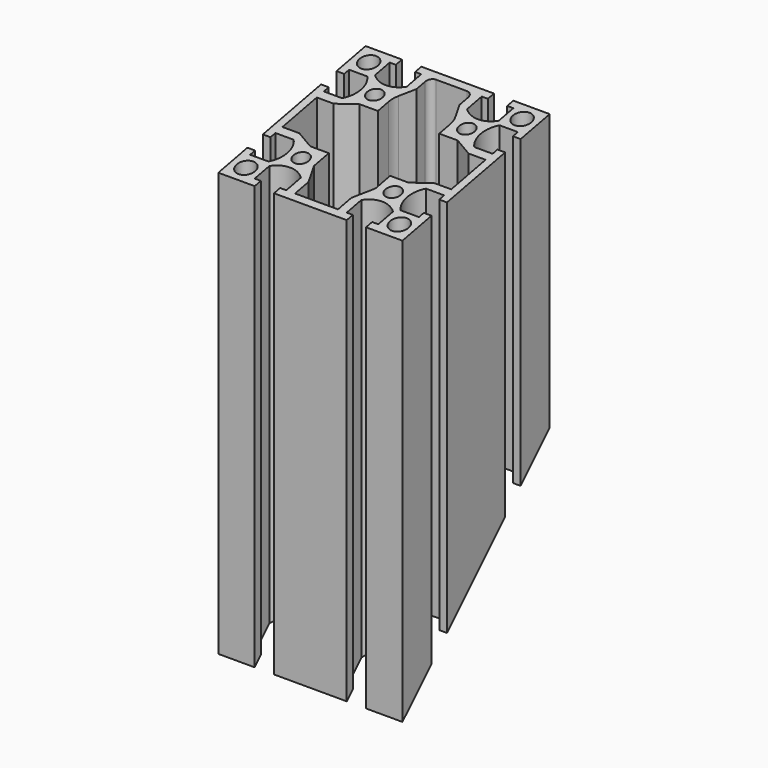
from build123d import *

# Parameters (mm, degrees)
F0_R          = 3
F0_R_2        = 2.5
F1_DEPTH      = 150
F2_R          = 2
F3_R          = 7
F6_DEPTH      = 30
F6_DEPTH_BACK = 30


# Not quite as in the source:
# - a feature names something its author has since deleted; it is built from what else it names


with BuildPart() as f1:
    # F0 (on Top) → F1 (new body)
    with BuildSketch(Plane.XY):
        with BuildLine():
            Line((18.15, -30), (30, -30))
            Line((30, -30), (30, -18.15))
            Line((30, -18.15), (27.5, -18.15))
            Line((27.5, -18.15), (27.5, -20.15))
            Line((27.5, -20.15), (21.5477069044, -20.15))
            ThreePointArc((21.5477069044, -20.15), (19.5, -15), (21.5477069044, -9.85))
            Line((21.5477069044, -9.85), (27.5, -9.85))
            Line((27.5, -9.85), (27.5, -11.85))
            Line((27.5, -11.85), (30, -11.85))
            Line((30, -11.85), (30, 11.85))
            Line((30, 11.85), (27.5, 11.85))
            Line((27.5, 11.85), (27.5, 9.85))
            Line((27.5, 9.85), (21.5477069044, 9.85))
            ThreePointArc((21.5477069044, 9.85), (19.5, 15), (21.5477069044, 20.15))
            Line((21.5477069044, 20.15), (27.5, 20.15))
            Line((27.5, 20.15), (27.5, 18.15))
            Line((27.5, 18.15), (30, 18.15))
            Line((30, 18.15), (30, 30))
            Line((30, 30), (18.15, 30))
            Line((18.15, 30), (18.15, 27.5))
            Line((18.15, 27.5), (20.15, 27.5))
            Line((20.15, 27.5), (20.15, 21.5477069044))
            ThreePointArc((20.15, 21.5477069044), (15, 19.5), (9.85, 21.5477069044))
            Line((9.85, 21.5477069044), (9.85, 27.5))
            Line((9.85, 27.5), (11.85, 27.5))
            Line((11.85, 27.5), (11.85, 30))
            Line((11.85, 30), (-11.85, 30))
            Line((-11.85, 30), (-11.85, 27.5))
            Line((-11.85, 27.5), (-9.85, 27.5))
            Line((-9.85, 27.5), (-9.85, 21.5477069044))
            ThreePointArc((-9.85, 21.5477069044), (-15, 19.5), (-20.15, 21.5477069044))
            Line((-20.15, 21.5477069044), (-20.15, 27.5))
            Line((-20.15, 27.5), (-18.15, 27.5))
            Line((-18.15, 27.5), (-18.15, 30))
            Line((-18.15, 30), (-30, 30))
            Line((-30, 30), (-30, 18.15))
            Line((-30, 18.15), (-27.5, 18.15))
            Line((-27.5, 18.15), (-27.5, 20.15))
            Line((-27.5, 20.15), (-21.5477069044, 20.15))
            ThreePointArc((-21.5477069044, 20.15), (-19.5, 15), (-21.5477069044, 9.85))
            Line((-21.5477069044, 9.85), (-27.5, 9.85))
            Line((-27.5, 9.85), (-27.5, 11.85))
            Line((-27.5, 11.85), (-30, 11.85))
            Line((-30, 11.85), (-30, -11.85))
            Line((-30, -11.85), (-27.5, -11.85))
            Line((-27.5, -11.85), (-27.5, -9.85))
            Line((-27.5, -9.85), (-21.5477069044, -9.85))
            ThreePointArc((-21.5477069044, -9.85), (-19.5, -15), (-21.5477069044, -20.15))
            Line((-21.5477069044, -20.15), (-27.5, -20.15))
            Line((-27.5, -20.15), (-27.5, -18.15))
            Line((-27.5, -18.15), (-30, -18.15))
            Line((-30, -18.15), (-30, -30))
            Line((-30, -30), (-18.15, -30))
            Line((-18.15, -30), (-18.15, -27.5))
            Line((-18.15, -27.5), (-20.15, -27.5))
            Line((-20.15, -27.5), (-20.15, -21.5477069044))
            ThreePointArc((-20.15, -21.5477069044), (-15, -19.5), (-9.85, -21.5477069044))
            Line((-9.85, -21.5477069044), (-9.85, -27.5))
            Line((-9.85, -27.5), (-11.85, -27.5))
            Line((-11.85, -27.5), (-11.85, -30))
            Line((-11.85, -30), (11.85, -30))
            Line((11.85, -30), (11.85, -27.5))
            Line((11.85, -27.5), (9.85, -27.5))
            Line((9.85, -27.5), (9.85, -21.5477069044))
            ThreePointArc((9.85, -21.5477069044), (15, -19.5), (20.15, -21.5477069044))
            Line((20.15, -21.5477069044), (20.15, -27.5))
            Line((20.15, -27.5), (18.15, -27.5))
            Line((18.15, -27.5), (18.15, -30))
        make_face()
        with Locations((-25, -25)):
            Circle(F0_R, mode=Mode.SUBTRACT)
        with Locations((-15, -15)):
            Circle(F0_R_2, mode=Mode.SUBTRACT)
        with Locations((25, -25)):
            Circle(F0_R, mode=Mode.SUBTRACT)
        with Locations((15, -15)):
            Circle(F0_R_2, mode=Mode.SUBTRACT)
        with Locations((-25, 25)):
            Circle(F0_R, mode=Mode.SUBTRACT)
        with Locations((-15, 15)):
            Circle(F0_R_2, mode=Mode.SUBTRACT)
        Polygon((-7, 22), (-7, 27.5), (0, 27.5), (7, 27.5), (7, 22), (10, 16), (10, 10), (16, 10), (22, 7), (27.5, 7), (27.5, 0), (27.5, -7), (22, -7), (16, -10), (10, -10), (10, -16), (7, -22), (7, -27.5), (0, -27.5), (-7, -27.5), (-7, -22), (-10, -16), (-10, -10), (-16, -10), (-22, -7), (-27.5, -7), (-27.5, 0), (-27.5, 7), (-22, 7), (-16, 10), (-10, 10), (-10, 16), align=None, mode=Mode.SUBTRACT)
        with Locations((15, 15)):
            Circle(F0_R_2, mode=Mode.SUBTRACT)
        with Locations((25, 25)):
            Circle(F0_R, mode=Mode.SUBTRACT)
    extrude(amount=F1_DEPTH)

    # F2
    f2_edges = [f1.edges().sort_by_distance(p)[0] for p in [
        (-7, 27.5, 75),
        (7, 27.5, 75),
    ]]
    fillet(f2_edges, radius=F2_R)

    # F3
    f3_edges = [f1.edges().sort_by_distance(p)[0] for p in [
        (-10, 16, 75),
        (10, 16, 75),
    ]]
    fillet(f3_edges, radius=F3_R)

    # F5 (on Right) → F6 (cut, two sides)
    with BuildSketch(Plane.YZ) as f6_sk:
        Polygon((115.2614038106, 44.5196963257), (64.8905500682, 94.8905500682), (-30, 0), (20.3708537424, -50.3708537424), align=None)
        Polygon((30, 150), (10.7683995954, 246.6837842107), (-148.7245392843, 214.9586661578), (-129.4929388797, 118.2748819471), align=None)
    extrude(amount=F6_DEPTH, mode=Mode.SUBTRACT)
    extrude(f6_sk.sketch, amount=-F6_DEPTH_BACK, mode=Mode.SUBTRACT)


solid = f1.part
